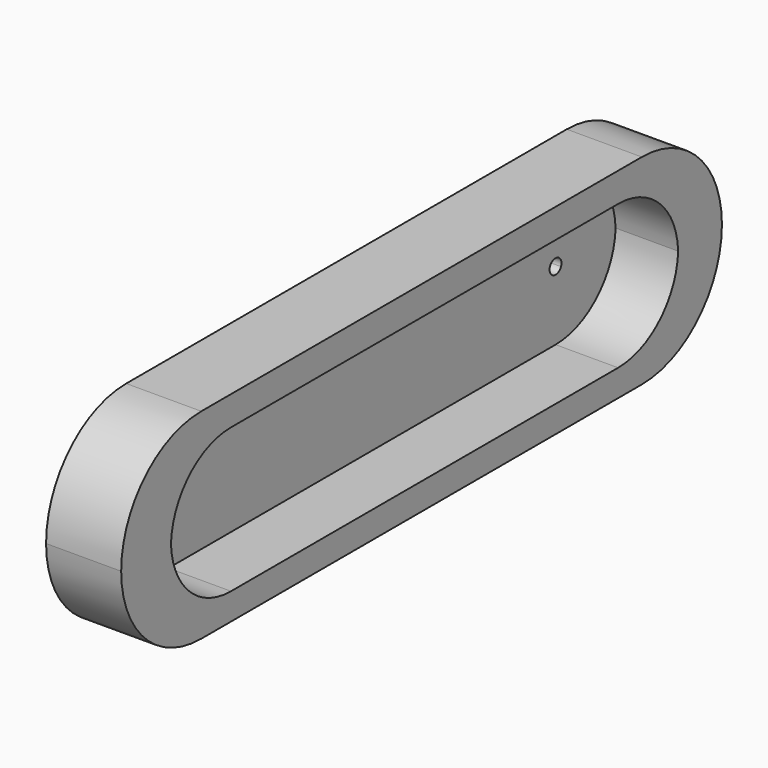
from build123d import *

# Parameters (mm, degrees)
F0_W        = 762
F0_H        = 203.2
F1_DEPTH    = 76.2
F2_R        = 101.59999
F3_W        = 643.4846520424
F3_H        = 146.4012786746
F4_DEPTH    = 63.5
F5_T1_DEPTH = 63.5
F8_DEPTH    = 25.4
F9_R        = 7.62
F10_DEPTH   = 25.4


# Not quite as in the source:
# - a fillet or chamfer that OpenCascade refuses, or shapes differently, is made with other operations: its cross-section is extruded or revolved along the edge and cut away or added
# - a fillet or chamfer is up to 0.001 mm smaller than in the source, because OpenCascade refuses the exact size


with BuildPart() as f1:
    # F0 (on Right) → F1 (new body)
    with BuildSketch(Plane.YZ):
        with Locations((20.2849134803, -13.820597699)):
            Rectangle(F0_W, F0_H)
    extrude(amount=F1_DEPTH)

    # F2 (radius 101.6 in the source; OpenCascade refuses exactly that, so slightly less here)
    f2_edges = [f1.edges().sort_by_distance(p)[0] for p in [
        (38.1, -360.715087, 87.779402),
        (38.1, -360.715087, -115.420598),
        (38.1, 401.284913, 87.779402),
        (38.1, 401.284913, -115.420598),
    ]]
    fillet(f2_edges, radius=F2_R)

    # F3 (on face) → F4 (cut)
    with BuildSketch(Plane.YZ.offset(76.2)):
        with Locations((24.1151750088, -15.0973536074)):
            Rectangle(F3_W, F3_H)
    extrude(amount=-F4_DEPTH, mode=Mode.SUBTRACT)

    # F5: fillet of radius 76.2 on 4 edges, made by hand

    # F5_s2 → F5_t1 (join)
    with BuildSketch(Plane.YZ.offset(12.7)):
        with BuildLine():
            ThreePointArc((-221.4271510124, 58.1032857299), (-275.3086877388, 35.7848224563), (-297.6271510124, -18.0967142701))
            Line((-297.6271510124, -18.0967142701), (-297.6271510124, 58.1032857299))
            Line((-297.6271510124, 58.1032857299), (-221.4271510124, 58.1032857299))
        make_face()
        with BuildLine():
            ThreePointArc((-297.6271510124, -12.0979929447), (-275.3086877388, -65.9795296711), (-221.4271510124, -88.2979929447))
            Line((-221.4271510124, -88.2979929447), (-297.6271510124, -88.2979929447))
            Line((-297.6271510124, -88.2979929447), (-297.6271510124, -12.0979929447))
        make_face()
        with BuildLine():
            ThreePointArc((269.65750103, 58.1032857299), (323.5390377564, 35.7848224563), (345.85750103, -18.0967142701))
            Line((345.85750103, -18.0967142701), (345.85750103, 58.1032857299))
            Line((345.85750103, 58.1032857299), (269.65750103, 58.1032857299))
        make_face()
        with BuildLine():
            ThreePointArc((269.65750103, -88.2979929447), (323.5390377564, -65.9795296711), (345.85750103, -12.0979929447))
            Line((345.85750103, -12.0979929447), (345.85750103, -88.2979929447))
            Line((345.85750103, -88.2979929447), (269.65750103, -88.2979929447))
        make_face()
    extrude(amount=F5_T1_DEPTH)

    # F7 (on face) → F8 (cut)
    with BuildSketch(Plane(origin=(0, 0, 0), x_dir=(0, -1, 0), z_dir=(-1, 0, 0))):
        with BuildLine():
            ThreePointArc((-276.6019562226, -21.4793750917), (-268.0456280954, -25.6827990477), (-262.0824047375, -18.2450916618))
            ThreePointArc((-262.0824047375, -18.2450916618), (-262.2195694481, -16.8057946003), (-262.6261254806, -15.4183140124))
            ThreePointArc((-262.6261254806, -15.4183140124), (-272.557495484, -11.6617121999), (-276.6019562226, -21.4793750917))
        make_face()
    extrude(amount=-F8_DEPTH, mode=Mode.SUBTRACT)

    # F9 (on face) → F10 (cut)
    with BuildSketch(Plane(origin=(0, 0, 0), x_dir=(0, -1, 0), z_dir=(-1, 0, 0))):
        with Locations((221.1862802505, -18.3496363461)):
            Circle(F9_R)
    extrude(amount=-F10_DEPTH, mode=Mode.SUBTRACT)


solid = f1.part
